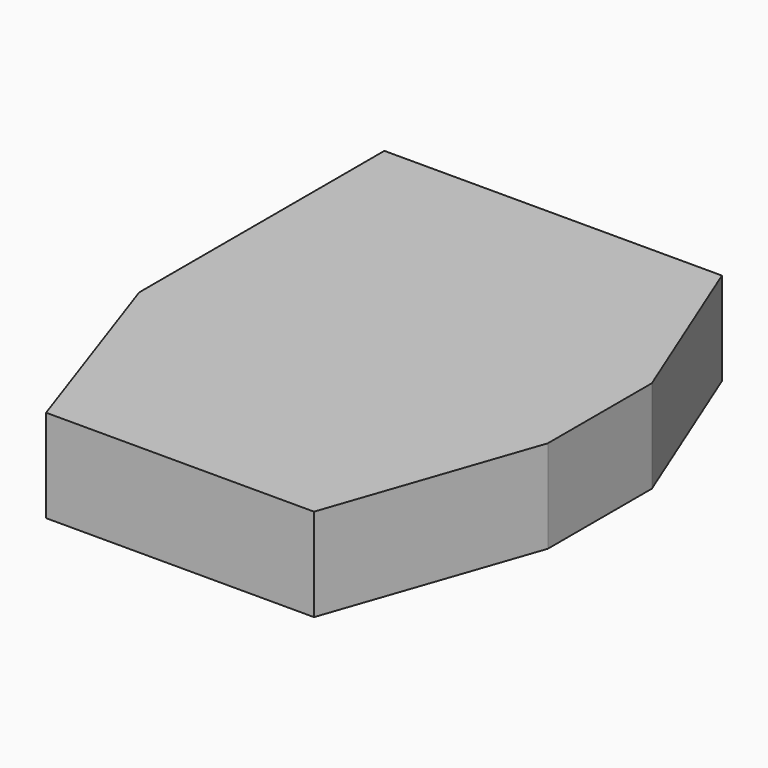
from build123d import *

# Parameters (mm, degrees)
F1_DEPTH = 127


# Not quite as in the source:
# - the program builds the solid bodies; features that only make, move or delete a surface that nothing else refers to are left out


with BuildPart() as f1:
    # F0 (on Top) → F1 (new body)
    with BuildSketch(Plane.XY):
        Polygon((-183.2191318646, -368.3), (183.2191318646, -368.3), (279.4, -88.9), (279.4, 88.9), (182.2553741554, 330.2), (-279.4, 330.2), (-279.4, 88.9), (-279.4, -88.9), align=None)
    extrude(amount=F1_DEPTH)


solid = f1.part
